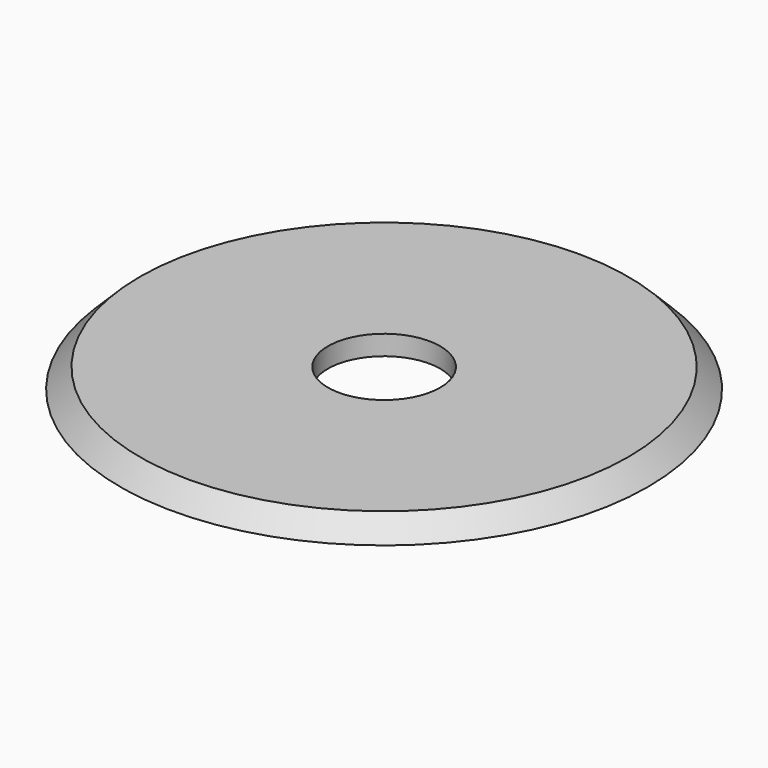
from build123d import *

# Parameters (mm, degrees)
F0_R     = 20
F0_R_2   = 4.25
F1_DEPTH = 1.5
F2_SIZE  = 1.49999


# Not quite as in the source:
# - a fillet or chamfer is up to 0.001 mm smaller than in the source, because OpenCascade refuses the exact size


with BuildPart() as f1:
    # F0 (on Top) → F1 (new body)
    with BuildSketch(Plane.XY):
        Circle(F0_R)
        Circle(F0_R_2, mode=Mode.SUBTRACT)
    extrude(amount=F1_DEPTH)

    # F2 (size 1.5 in the source; OpenCascade refuses exactly that, so slightly less here)
    f2_edges = [f1.edges().sort_by_distance(p)[0] for p in [
        (-20, 0, 1.5),
    ]]
    chamfer(f2_edges, length=F2_SIZE)


solid = f1.part
